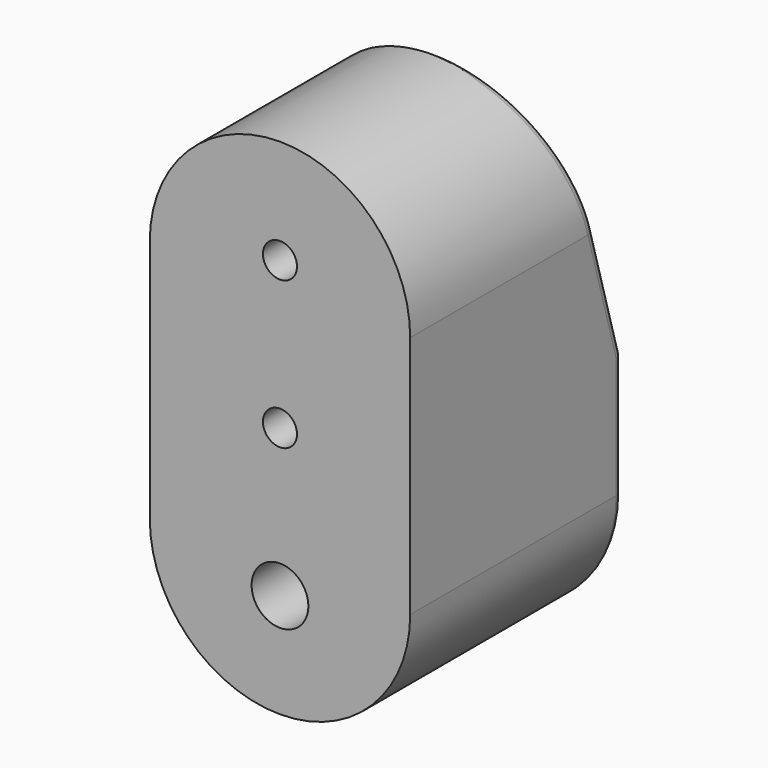
from build123d import *

# Parameters (mm, degrees)
F0_R          = 3.75
F0_R_2        = 2.25
F1_DEPTH      = 10
F1_DEPTH_BACK = 5
F4_DEPTH      = 1.9
F5_DEPTH      = 5
F7_DEPTH      = 20
F8_W          = 32.4212387204
F8_H          = 10.9641202658
F9_DEPTH      = 20
F10_R         = 3.75
F11_DEPTH     = 16.2
F12_S5_R      = 3.75
F12_T6_DEPTH  = 8
F13_S6_R      = 3.75
F13_T7_DEPTH  = 8
F13_S13_R     = 3.75
F13_T14_DEPTH = 8
F13_S20_R     = 3.75
F13_T21_DEPTH = 8
F14_R         = 1
F16_DEPTH     = 25
F17_DEPTH     = 22


# Not quite as in the source:
# - a fillet or chamfer that OpenCascade refuses, or shapes differently, is made with other operations: its cross-section is extruded or revolved along the edge and cut away or added


with BuildPart() as f1:
    # F0 (on Front) → F1 (new body, two sides)
    with BuildSketch(Plane.XZ) as f1_sk:
        with BuildLine():
            Line((-17.2, 16.1), (-17.2, -16.1))
            ThreePointArc((-17.2, -16.1), (0, -33.3), (17.2, -16.1))
            Line((17.2, -16.1), (17.2, 16.1))
            ThreePointArc((17.2, 16.1), (0, 33.3), (-17.2, 16.1))
        make_face()
        with Locations((0, -19.5)):
            Circle(F0_R, mode=Mode.SUBTRACT)
        Circle(F0_R_2, mode=Mode.SUBTRACT)
        with Locations((0, 19.5)):
            Circle(F0_R_2, mode=Mode.SUBTRACT)
    extrude(amount=-F1_DEPTH)
    extrude(f1_sk.sketch, amount=F1_DEPTH_BACK)

    # F2 (on Front) → F4 (cut)
    with BuildSketch(Plane.XZ):
        Polygon((-8.88, -33.3), (0, -33.3), (8.88, -33.3), (8.45, -11.4), (8.45, 0), (0, 0), (-8.45, 0), (-8.45, -11.4), align=None)
    extrude(amount=-F4_DEPTH, mode=Mode.SUBTRACT)

    # F3 (on Front) → F5 (cut)
    with BuildSketch(Plane.XZ):
        Polygon((-6.3, -34.5453813779), (0, -34.5453813779), (6.3, -34.5453813779), (6.3, 0), (0, 0), (-6.3, 0), align=None)
    extrude(amount=-F5_DEPTH, mode=Mode.SUBTRACT)

    # F6 (on Right) → F7 (cut, symmetric)
    with BuildSketch(Plane.YZ):
        Polygon((-8.5170516447, 64.5766333631), (10, 0), (10, 64.5766333631), align=None)
    extrude(amount=F7_DEPTH, both=True, mode=Mode.SUBTRACT)

    # F8 (on Right) → F9 (cut, symmetric)
    with BuildSketch(Plane.YZ):
        with Locations((6.0222381726, -36.4180710167)):
            Rectangle(F8_W, F8_H)
    extrude(amount=F9_DEPTH, both=True, mode=Mode.SUBTRACT)

    # F10 (on Front) → F11 (cut)
    with BuildSketch(Plane.XZ):
        Circle(F10_R)
        with Locations((0, 19.4826573133)):
            Circle(F10_R)
    extrude(amount=-F11_DEPTH, mode=Mode.SUBTRACT)

    # F12: chamfer of 2.5 on 1 edges, made by hand


with BuildPart() as f12_tool2:
    # F12_s3 → F12_t4 (revolve)
    with BuildSketch(Plane.XY.offset(19.5)):
        Polygon((2.25, -2.5), (4.75, 0), (2.25, 0), align=None)
    revolve(axis=Axis((0, 0, 19.5), (0, -1, 0)))

    # F12_s5 → F12_t6 (intersect, symmetric)
    with BuildSketch(Plane.XZ.offset(1.2)):
        with Locations((0, 19.4826573133)):
            Circle(F12_S5_R)
    extrude(amount=F12_T6_DEPTH, both=True, mode=Mode.INTERSECT)


with BuildPart() as f1_1:
    add(f1.part)

    # F12_t1: cut F12_tool2
    add(f12_tool2.part, mode=Mode.SUBTRACT)

    # F13: chamfer of 2.5 on 1 edges, made by hand


with BuildPart() as f13_tool2:
    # F13_s3 → F13_t4 (revolve)
    with BuildSketch(Plane.XY):
        Polygon((4.75, 0), (2.25, -2.5), (2.25, 0), align=None)
    revolve(axis=Axis((0, 0, 0), (0, 1, 0)))

    split(bisect_by=Plane.XY, keep=Keep.BOTTOM)

    # F13_s6 → F13_t7 (cut, symmetric)
    with BuildSketch(Plane.XZ.offset(1.2)):
        Circle(F13_S6_R)
    extrude(amount=F13_T7_DEPTH, both=True, mode=Mode.SUBTRACT)


with BuildPart() as f1_2:
    add(f1_1.part)

    # F13_t1: cut F13_tool2
    add(f13_tool2.part, mode=Mode.SUBTRACT)


with BuildPart() as f13_tool9:
    # F13_s10 → F13_t11 (revolve)
    with BuildSketch(Plane.XY):
        Polygon((4.75, 0), (2.25, -2.5), (2.25, 0), align=None)
    revolve(axis=Axis((0, 0, 0), (0, 1, 0)))

    split(bisect_by=Plane.XY, keep=Keep.BOTTOM)

    # F13_s13 → F13_t14 (intersect, symmetric)
    with BuildSketch(Plane.XZ.offset(1.2)):
        Circle(F13_S13_R)
    extrude(amount=F13_T14_DEPTH, both=True, mode=Mode.INTERSECT)


with BuildPart() as f1_3:
    add(f1_2.part)

    # F13_t8: cut F13_tool9
    add(f13_tool9.part, mode=Mode.SUBTRACT)


with BuildPart() as f13_tool16:
    # F13_s17 → F13_t18 (revolve)
    with BuildSketch(Plane.XY):
        Polygon((4.75, 0), (2.25, -2.5), (2.25, 0), align=None)
    revolve(axis=Axis((0, 0, 0), (0, 1, 0)))

    split(bisect_by=Plane.XY, keep=Keep.TOP)

    # F13_s20 → F13_t21 (intersect, symmetric)
    with BuildSketch(Plane.XZ.offset(1.2)):
        Circle(F13_S20_R)
    extrude(amount=F13_T21_DEPTH, both=True, mode=Mode.INTERSECT)


with BuildPart() as f1_4:
    add(f1_3.part)

    # F13_t15: cut F13_tool16
    add(f13_tool16.part, mode=Mode.SUBTRACT)

    # F14
    f14_edges = [f1_4.edges().sort_by_distance(p)[0] for p in [
        (-17.2, 7.6917, 8.05),
        (0, 0.451379, 33.3),
        (17.2, 7.6917, 8.05),
        (17.2, 10, -8.05),
        (14.925185, 10, -24.648617),
        (-14.925185, 10, -24.648617),
        (-17.2, 10, -8.05),
        (0, 10, -30.936011),
    ]]
    fillet(f14_edges, radius=F14_R)

    # F0 (on Front) → F16 (join)
    with BuildSketch(Plane.XZ):
        with BuildLine():
            Line((-17.2, 16.1), (-17.2, -16.1))
            ThreePointArc((-17.2, -16.1), (0, -33.3), (17.2, -16.1))
            Line((17.2, -16.1), (17.2, 16.1))
            ThreePointArc((17.2, 16.1), (0, 33.3), (-17.2, 16.1))
        make_face()
        with Locations((0, -19.5)):
            Circle(F0_R, mode=Mode.SUBTRACT)
        Circle(F0_R_2, mode=Mode.SUBTRACT)
        with Locations((0, 19.5)):
            Circle(F0_R_2, mode=Mode.SUBTRACT)
    extrude(amount=F16_DEPTH)

    # F0 (on Front) → F17 (cut)
    with BuildSketch(Plane.XZ):
        with Locations((0, -19.5)):
            Circle(F0_R)
        with Locations((0, -19.5)):
            Circle(F0_R_2, mode=Mode.SUBTRACT)
    extrude(amount=F17_DEPTH, mode=Mode.SUBTRACT)


solid = f1_4.part
